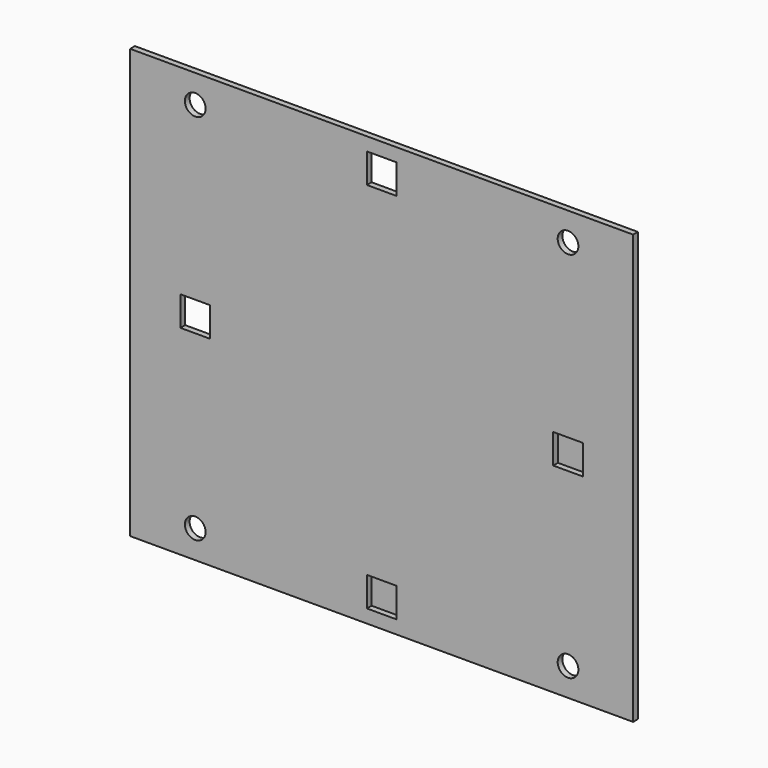
from build123d import *

# Parameters (mm, degrees)
F0_W     = 10
F0_H     = 10
F7_DEPTH = 20
F8_DEPTH = 20
F0_W_2   = 170
F0_H_2   = 145
F0_R     = 3.5
F9_DEPTH = 2


# Not quite as in the source:
# - the program builds the solid bodies; features that only make, move or delete a surface that nothing else refers to are left out


with BuildPart() as f7:
    # F0 (on Front) → F7 (new body)
    with BuildSketch(Plane.XZ):
        with Locations((34.6195249557, 23.5447047651)):
            Rectangle(F0_W, F0_H)
    extrude(amount=-F7_DEPTH)


with BuildPart() as f8:
    # F0 (on Front) → F8 (new body)
    with BuildSketch(Plane.XZ):
        with Locations((-28.3804750443, -39.4552952349)):
            Rectangle(F0_W, F0_H)
    extrude(amount=-F8_DEPTH)


with BuildPart() as f9:
    # F0 (on Front) → F9 (new body)
    with BuildSketch(Plane.XZ):
        with Locations((-28.3804750443, 23.5447047651)):
            Rectangle(F0_W_2, F0_H_2)
        with Locations((-91.3804750443, -39.4552952349)):
            Circle(F0_R, mode=Mode.SUBTRACT)
        with Locations((-28.3804750443, -39.4552952349)):
            Rectangle(F0_W, F0_H, mode=Mode.SUBTRACT)
        with Locations((34.6195249557, -39.4552952349)):
            Circle(F0_R, mode=Mode.SUBTRACT)
        with Locations((-91.3804750443, 23.5447047651)):
            Rectangle(F0_W, F0_H, mode=Mode.SUBTRACT)
        with Locations((-91.3804750443, 86.5447047651)):
            Circle(F0_R, mode=Mode.SUBTRACT)
        with Locations((34.6195249557, 23.5447047651)):
            Rectangle(F0_W, F0_H, mode=Mode.SUBTRACT)
        with Locations((-28.3804750443, 86.5447047651)):
            Rectangle(F0_W, F0_H, mode=Mode.SUBTRACT)
        with Locations((34.6195249557, 86.5447047651)):
            Circle(F0_R, mode=Mode.SUBTRACT)
    extrude(amount=F9_DEPTH)


solid = Compound([f7.part, f8.part, f9.part])
